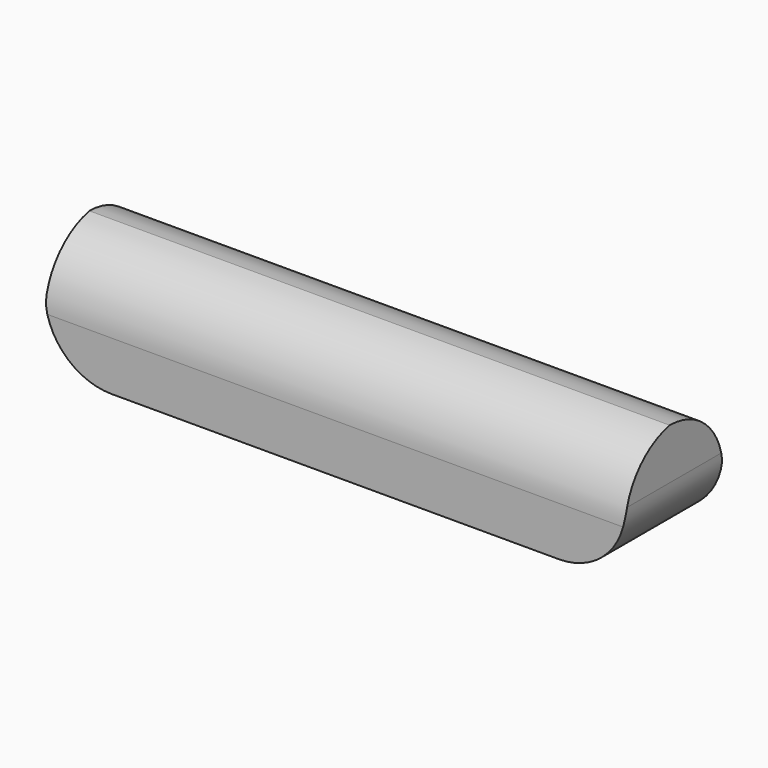
from build123d import *

# Parameters (mm, degrees)
F0_W        = 49.567822367
F0_H        = 20.8045206964
F1_DEPTH    = 20
F2_R        = 11.3468037432
F3_T1_DEPTH = 107.5148856448
F4_R        = 11.3468037432


# Not quite as in the source:
# - a fillet or chamfer that OpenCascade refuses, or shapes differently, is made with other operations: its cross-section is extruded or revolved along the edge and cut away or added


with BuildPart() as f1:
    # F0 (on Top) → F1 (new body)
    with BuildSketch(Plane.XY):
        with Locations((-24.7839111835, -10.4022603482)):
            Rectangle(F0_W, F0_H)
    extrude(amount=F1_DEPTH)

    # F2
    f2_edges = [f1.edges().sort_by_distance(p)[0] for p in [
        (-24.783911, 0, 20),
    ]]
    fillet(f2_edges, radius=F2_R)

    # F3: fillet of radius 11.8296464556 on 1 edges, made by hand

    # F3_s2 → F3_t1 (cut)
    with BuildSketch(Plane.YZ.offset(-78.5413540059)):
        with BuildLine():
            ThreePointArc((-11.3468037432, 20), (-18.1400153389, 15.8899405195), (-20.8045206964, 8.4105873444))
            Line((-20.8045206964, 8.4105873444), (-20.8045206964, 20))
            Line((-20.8045206964, 20), (-11.3468037432, 20))
        make_face()
    extrude(amount=F3_T1_DEPTH, mode=Mode.SUBTRACT)

    # F4
    f4_edges = [f1.edges().sort_by_distance(p)[0] for p in [
        (-49.567822, -10.40226, 0),
    ]]
    fillet(f4_edges, radius=F4_R)

    # F5: F1 across face


with BuildPart() as f1_1:
    add(f1.part)
    add(f1.part.mirror(Plane(origin=(0, -10.3947828822, 8.8652235267), x_dir=(0, 1, 0), z_dir=(1, 0, 0))))


solid = f1_1.part
